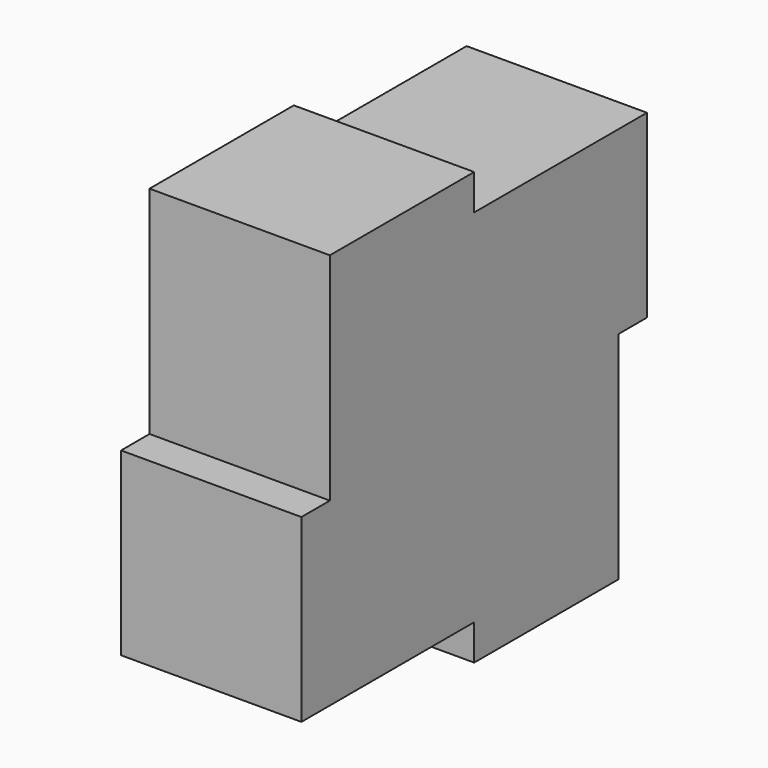
from build123d import *

# Parameters (mm, degrees)
F0_W     = 76
F0_H     = 76
F1_DEPTH = 91
F2_COUNT = 4


with BuildPart() as f1:
    # F0 (on Top) → F1 (new body)
    with BuildSketch(Plane.XY):
        with Locations((-38, 38)):
            Rectangle(F0_W, F0_H)
    extrude(amount=F1_DEPTH)

    # F2: F1 ×4 about axis
    f2_axis = Axis((-38, 0, 91), (1, 0, 0))


with BuildPart() as f1_1:
    add(f1.part)
    for i in range(1, F2_COUNT):
        add(f1.part.rotate(f2_axis, i * 360 / F2_COUNT))


solid = f1_1.part
